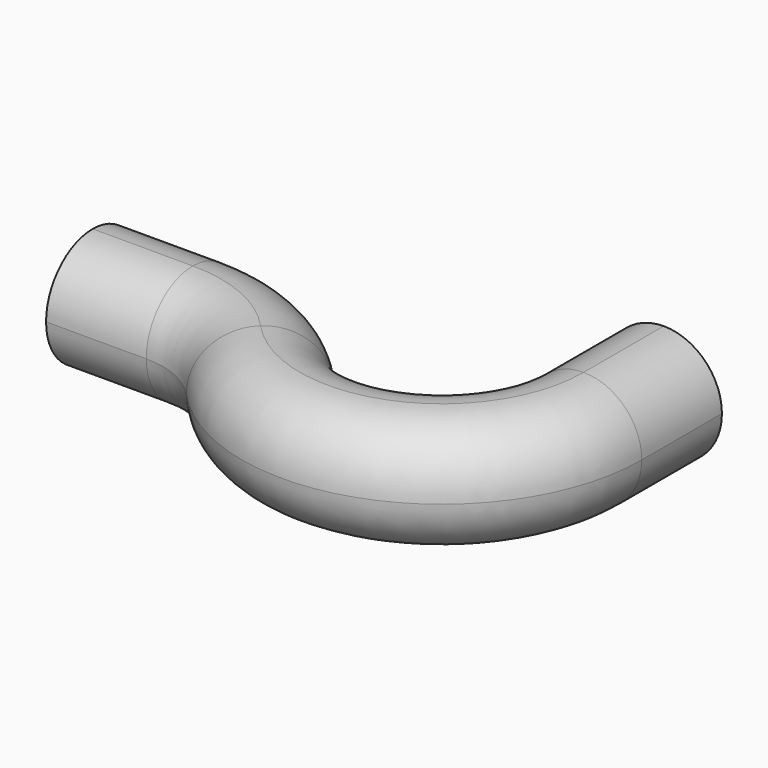
from build123d import *

# Parameters (mm, degrees)
F1_W = 3.683
F1_H = 3.683
F1_R = 1.5875
F3_R = 1.84149


# Not quite as in the source:
# - a fillet or chamfer is up to 0.001 mm smaller than in the source, because OpenCascade refuses the exact size


with BuildPart() as f2:
    # F2: sweep along a path in F0
    with BuildLine(Plane.XY) as f2_path:
        Line((0, 0), (0, -3.175))
        ThreePointArc((0, -3.175), (-2.8623663141, -7.3624320102), (-7.8033180665, -6.2158180665))
        ThreePointArc((-7.8033180665, -6.2158180665), (-9.3053739342, -5.1418390585), (-11.1125, -4.7625))
        Line((-11.1125, -4.7625), (-14.2875, -4.7625))
    # F1 (on Front) → F2 (sweep)
    with BuildSketch(Plane.XZ):
        Rectangle(F1_W, F1_H)
        Circle(F1_R, mode=Mode.SUBTRACT)
    sweep(path=f2_path.line)

    # F3 (radius 1.8415 in the source; OpenCascade refuses exactly that, so slightly less here)
    f3_edges = [f2.edges().sort_by_distance(p)[0] for p in [
        (-12.7, -6.604, -1.8415),
        (-12.7, -6.604, 1.8415),
        (-12.7, -2.921, 1.8415),
        (-12.7, -2.921, -1.8415),
    ]]
    fillet(f3_edges, radius=F3_R)


solid = f2.part
